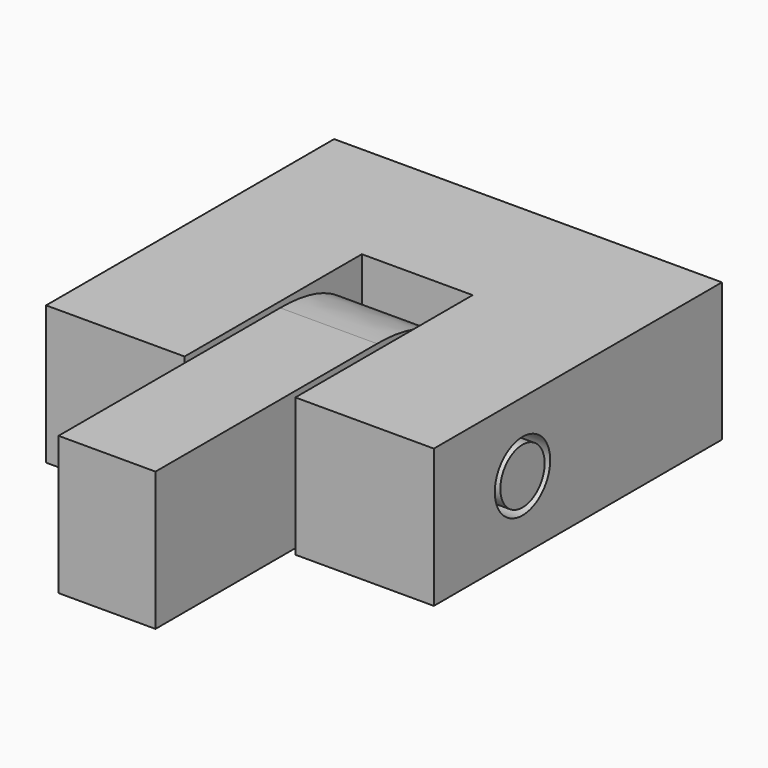
from build123d import *

# Parameters (mm, degrees)
F1_DEPTH    = 12.7
F2_R        = 3.175
F3_DEPTH    = 50.8
F4_W        = 8.89
F4_H        = 35.56
F5_DEPTH    = 12.7
F6_R        = 2.54
F7_DEPTH    = 35.56
F8_T1_DEPTH = 59.69


# Not quite as in the source:
# - a fillet or chamfer that OpenCascade refuses, or shapes differently, is made with other operations: its cross-section is extruded or revolved along the edge and cut away or added


with BuildPart() as f1:
    # F0 (on Top) → F1 (new body)
    with BuildSketch(Plane.XY):
        Polygon((-10.16, 0), (0, 0), (0, -20.32), (12.7, -20.32), (12.7, 12.7), (-22.86, 12.7), (-22.86, -20.32), (-10.16, -20.32), align=None)
    extrude(amount=F1_DEPTH)

    # F2 (on face) → F3 (cut)
    with BuildSketch(Plane(origin=(-22.86, 0, 0), x_dir=(0, -1, 0), z_dir=(-1, 0, 0))):
        with Locations((10.16, 6.35)):
            Circle(F2_R)
    extrude(amount=-F3_DEPTH, mode=Mode.SUBTRACT)


with BuildPart() as f5:
    # F4 (on Top) → F5 (new body)
    with BuildSketch(Plane.XY):
        with Locations((-5.08, -17.78)):
            Rectangle(F4_W, F4_H)
    extrude(amount=F5_DEPTH)

    # F6 (on face) → F7 (join)
    with BuildSketch(Plane(origin=(-22.86, 0, 0), x_dir=(0, -1, 0), z_dir=(-1, 0, 0))):
        with Locations((10.16, 6.35)):
            Circle(F6_R)
    extrude(amount=-F7_DEPTH)

    # F8: fillet of radius 10.16 on 2 edges, made by hand

    # F8_s2 → F8_t1 (cut)
    with BuildSketch(Plane.YZ.offset(-34.925)):
        with BuildLine():
            add(Edge.make_bspline(
                [(-10.16, 12.7), (0, 12.7), (0, 2.54)],
                knots=[0, 0, 0, 1, 1, 1], degree=2, weights=[1, 1, 1]))
            Line((0, 2.54), (0, 12.7))
            Line((0, 12.7), (-10.16, 12.7))
        make_face()
        with BuildLine():
            add(Edge.make_bspline(
                [(-10.16, 0), (0, 0), (0, 10.16)],
                knots=[0, 0, 0, 1, 1, 1], degree=2, weights=[1, 1, 1]))
            Line((0, 10.16), (0, 0))
            Line((0, 0), (-10.16, 0))
        make_face()
    extrude(amount=F8_T1_DEPTH, mode=Mode.SUBTRACT)


solid = Compound([f1.part, f5.part])
